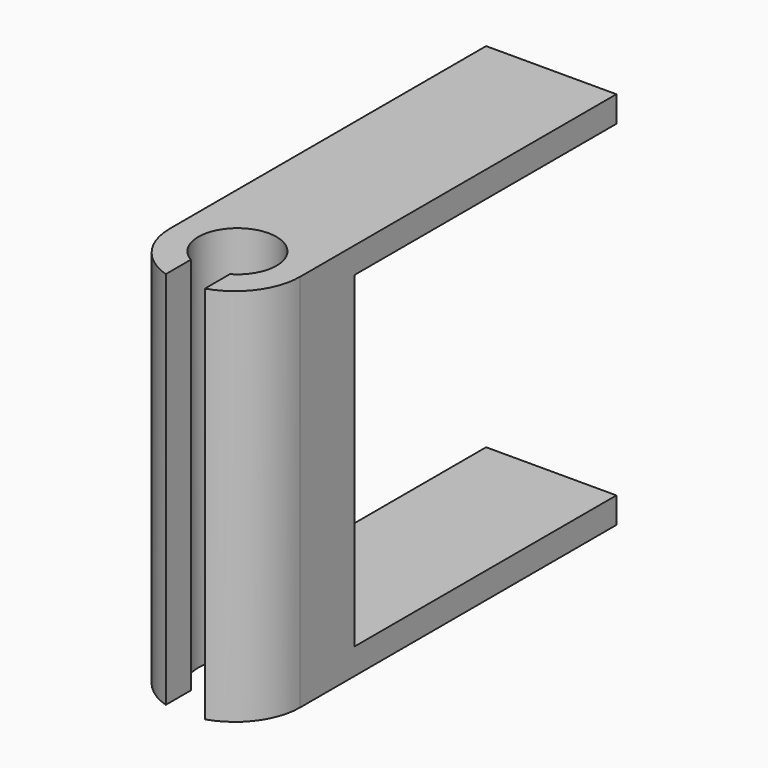
from build123d import *

# Parameters (mm, degrees)
F3_W        = 10
F3_H        = 25.1
F4_DEPTH    = 29.1
F5_DEPTH    = 27.1
F6_DEPTH    = 2
F7_T1_DEPTH = 52.9484800354


# Not quite as in the source:
# - a fillet or chamfer that OpenCascade refuses, or shapes differently, is made with other operations: its cross-section is extruded or revolved along the edge and cut away or added


with BuildPart() as f4:
    # F3 (on Top) → F4 (new body)
    with BuildSketch(Plane.XY):
        Rectangle(F3_W, F3_H)
        with BuildLine():
            Line((5, -12.55), (-5, -12.55))
            Line((-5, -12.55), (-5, -22.55))
            Line((-5, -22.55), (-1.5, -22.55))
            Line((-1.5, -22.55), (-1.5, -20.1480762114))
            ThreePointArc((-1.5, -20.1480762114), (0, -14.55), (1.5, -20.1480762114))
            Line((1.5, -20.1480762114), (1.5, -22.55))
            Line((1.5, -22.55), (5, -22.55))
            Line((5, -22.55), (5, -12.55))
        make_face()
    extrude(amount=F4_DEPTH)

    # F3 (on Top) → F5 (cut)
    with BuildSketch(Plane.XY):
        Rectangle(F3_W, F3_H)
    extrude(amount=F5_DEPTH, mode=Mode.SUBTRACT)

    # F3 (on Top) → F6 (join)
    with BuildSketch(Plane.XY):
        Rectangle(F3_W, F3_H)
        with BuildLine():
            Line((5, -12.55), (-5, -12.55))
            Line((-5, -12.55), (-5, -22.55))
            Line((-5, -22.55), (-1.5, -22.55))
            Line((-1.5, -22.55), (-1.5, -20.1480762114))
            ThreePointArc((-1.5, -20.1480762114), (0, -14.55), (1.5, -20.1480762114))
            Line((1.5, -20.1480762114), (1.5, -22.55))
            Line((1.5, -22.55), (5, -22.55))
            Line((5, -22.55), (5, -12.55))
        make_face()
    extrude(amount=F6_DEPTH)

    # F7: fillet of radius 5 on 2 edges, made by hand

    # F7_s2 → F7_t1 (cut)
    with BuildSketch(Plane.XY.offset(-11.9242400177)):
        with BuildLine():
            ThreePointArc((-1.5, -22.55), (-4.0311288741, -20.7383438845), (-5, -17.7803039929))
            Line((-5, -17.7803039929), (-5, -22.55))
            Line((-5, -22.55), (-1.5, -22.55))
        make_face()
        with BuildLine():
            ThreePointArc((5, -17.7803039929), (4.0311288741, -20.7383438845), (1.5, -22.55))
            Line((1.5, -22.55), (5, -22.55))
            Line((5, -22.55), (5, -17.7803039929))
        make_face()
    extrude(amount=F7_T1_DEPTH, mode=Mode.SUBTRACT)


solid = f4.part
